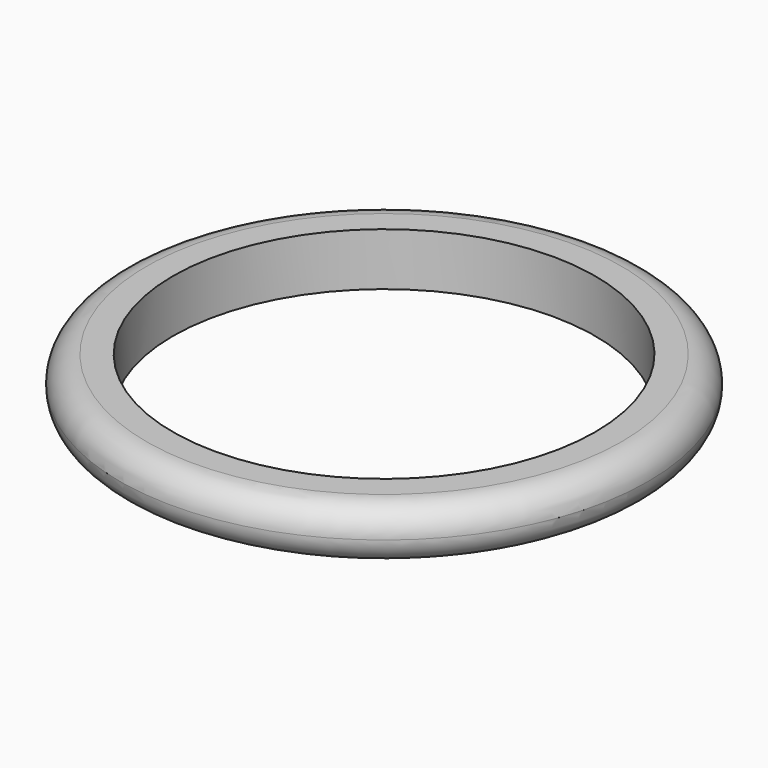
from build123d import *

# Parameters (mm, degrees)
F0_R     = 127
F0_R_2   = 101.6
F1_DEPTH = 25.4
F2_R     = 12.69999


# Not quite as in the source:
# - a fillet or chamfer is up to 0.001 mm smaller than in the source, because OpenCascade refuses the exact size


with BuildPart() as f1:
    # F0 (on Top) → F1 (new body)
    with BuildSketch(Plane.XY):
        Circle(F0_R)
        Circle(F0_R_2, mode=Mode.SUBTRACT)
    extrude(amount=-F1_DEPTH)

    # F2 (radius 12.7 in the source; OpenCascade refuses exactly that, so slightly less here)
    f2_edges = [f1.edges().sort_by_distance(p)[0] for p in [
        (-127, 0, 0),
        (-127, 0, -25.4),
    ]]
    fillet(f2_edges, radius=F2_R)


solid = f1.part
